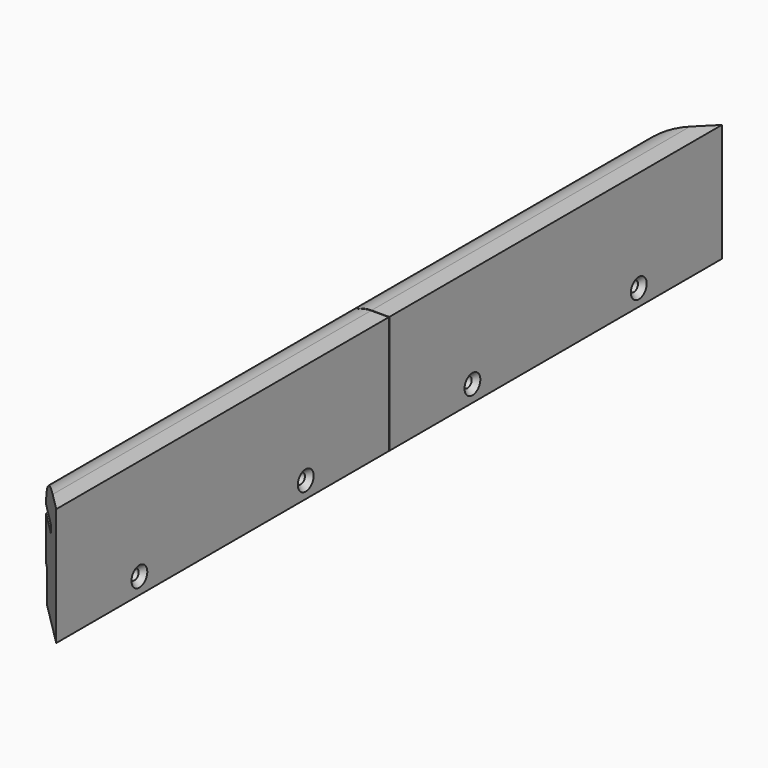
from build123d import *

# Parameters (mm, degrees)
F0_W            = 20
F0_H            = 46.5
F1_DEPTH        = 164
F2_W            = 164
F2_H            = 3.1
F3_DEPTH        = 10
F4_W            = 164
F4_H            = 13
F5_DEPTH        = 2
F7_DEPTH        = 46.5
F8_R            = 12.99999
F10_D           = 4
F10_DEPTH       = 20
F10_CSINK_D     = 7.8
F10_CSINK_ANGLE = 90
F10_TIP         = 1.2017212381


# Not quite as in the source:
# - a fillet or chamfer is up to 0.001 mm smaller than in the source, because OpenCascade refuses the exact size


with BuildPart() as f1:
    # F0 (on Front) → F1 (new body)
    with BuildSketch(Plane.XZ):
        Rectangle(F0_W, F0_H)
    extrude(amount=F1_DEPTH)

    # F2 (on face) → F3 (cut)
    with BuildSketch(Plane(origin=(-10, 0, 0), x_dir=(0, -1, 0), z_dir=(-1, 0, 0))):
        with Locations((82, 8.7)):
            Rectangle(F2_W, F2_H)
    extrude(amount=-F3_DEPTH, mode=Mode.SUBTRACT)

    # F4 (on face) → F5 (cut)
    with BuildSketch(Plane(origin=(-10, 0, 0), x_dir=(0, -1, 0), z_dir=(-1, 0, 0))):
        with Locations((82, -16.75)):
            Rectangle(F4_W, F4_H)
    extrude(amount=-F5_DEPTH, mode=Mode.SUBTRACT)

    # F6 (on face) → F7 (cut, through all)
    with BuildSketch(Plane.XY.offset(23.25)):
        Polygon((-10, 0), (-10, -20), (10, 0), align=None)
    extrude(amount=-F7_DEPTH, mode=Mode.SUBTRACT)

    # F8 (radius 13 in the source; OpenCascade refuses exactly that, so slightly less here)
    f8_edges = [f1.edges().sort_by_distance(p)[0] for p in [
        (-10, -92, 23.25),
    ]]
    fillet(f8_edges, radius=F8_R)

    # F10
    with Locations(Plane.YZ.offset(10)):
        with Locations((-123, -16.75), (-41, -16.75)):
            CounterSinkHole(F10_D / 2, F10_CSINK_D / 2, depth=F10_DEPTH, counter_sink_angle=F10_CSINK_ANGLE)
            with Locations((0, 0, -(F10_DEPTH + F10_TIP / 2))):  # 118° drill point
                Cone(0, F10_D / 2, F10_TIP, mode=Mode.SUBTRACT)


with BuildPart() as f12_1:
    # F12: instance of F1
    add(f1.part.mirror(Plane(origin=(0.7724850415, -164.1, -0.683742713), x_dir=(1, 0, 0), z_dir=(0, -1, 0))))


solid = Compound([f1.part, f12_1.part])
